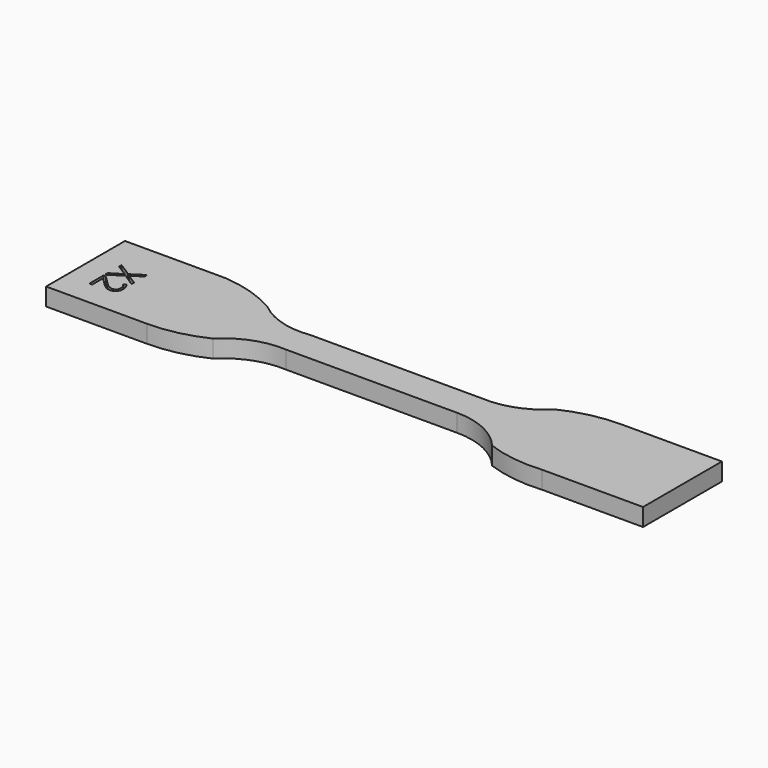
from build123d import *

# Parameters (mm, degrees)
F1_DEPTH     = 3.4
F2_TEXT_SIZE = 7.0564552314
F3_DEPTH     = 1


# Not quite as in the source:
# - Text() gives the source's letters only with a copy of the font that has no kerning and outlines rounded to 1/6400 em; it was checked with that copy


with BuildPart() as f1:
    # F0 (on Top) → F1 (new body)
    with BuildSketch(Plane.XY):
        with BuildLine():
            Line((-14.4320548165, 19.7811394548), (-33.8720548165, 19.7811394548))
            Line((-33.8720548165, 19.7811394548), (-33.8720548165, 0.7811394548))
            Line((-33.8720548165, 0.7811394548), (-14.4320548165, 0.7811394548))
            ThreePointArc((-14.4320548165, 0.7811394548), (-8.9053122052, 1.3996892086), (-3.6520548165, 3.2247301661))
            ThreePointArc((-3.6520548165, 3.2247301661), (1.3014698263, 6.4128780055), (7.1279451835, 7.2811394548))
            Line((7.1279451835, 7.2811394548), (40.1279451835, 7.2811394548))
            ThreePointArc((40.1279451835, 7.2811394548), (46.0837574042, 5.9511158081), (50.9079451835, 2.2137538538))
            ThreePointArc((50.9079451835, 2.2137538538), (56.2191047011, 0.9041953221), (61.6879451835, 0.7811394548))
            Line((61.6879451835, 0.7811394548), (81.1279451835, 0.7811394548))
            Line((81.1279451835, 0.7811394548), (81.1279451835, 19.7811394548))
            Line((81.1279451835, 19.7811394548), (61.6879451835, 19.7811394548))
            ThreePointArc((61.6879451835, 19.7811394548), (56.1612025723, 19.162589701), (50.9079451835, 17.3375487435))
            ThreePointArc((50.9079451835, 17.3375487435), (45.9544205407, 14.1494009041), (40.1279451835, 13.2811394548))
            Line((40.1279451835, 13.2811394548), (7.1279451835, 13.2811394548))
            ThreePointArc((7.1279451835, 13.2811394548), (1.4167452884, 13.6925537245), (-3.6520548165, 16.3560723447))
            ThreePointArc((-3.6520548165, 16.3560723447), (-8.8458057958, 18.686276846), (-14.4320548165, 19.7811394548))
        make_face()
    extrude(amount=F1_DEPTH)

    # F2 (on face) → F3 (cut)
    with BuildSketch(Plane.XY.offset(3.4)):
        with Locations(Location((-29.3720550835, 13.353464842), (0, 0, -90))):
            Text('X2', F2_TEXT_SIZE, font='Open Sans', text_align=(TextAlign.LEFT, TextAlign.BOTTOM))
    extrude(amount=-F3_DEPTH, mode=Mode.SUBTRACT)


solid = f1.part
